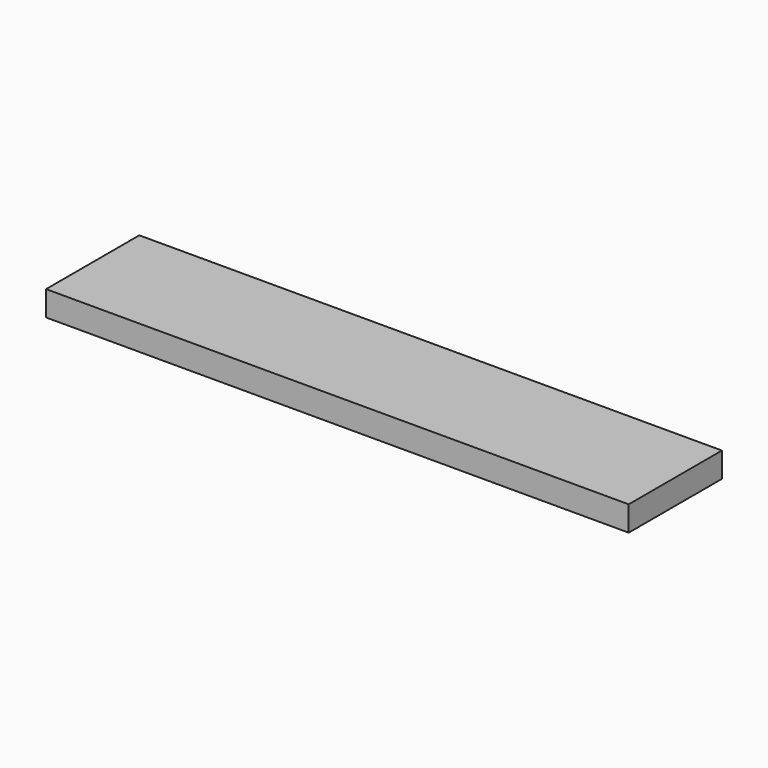
from build123d import *

# Parameters (mm, degrees)
F0_W     = 444.5
F0_H     = 88.9
F1_DEPTH = 19.05


# Not quite as in the source:
# - a feature of the source that left no trace in its solid (it failed there, or was rolled back) is left out


with BuildPart() as f1:
    # F0 (on Top) → F1 (new body)
    with BuildSketch(Plane.XY):
        Rectangle(F0_W, F0_H)
    extrude(amount=F1_DEPTH)


solid = f1.part
